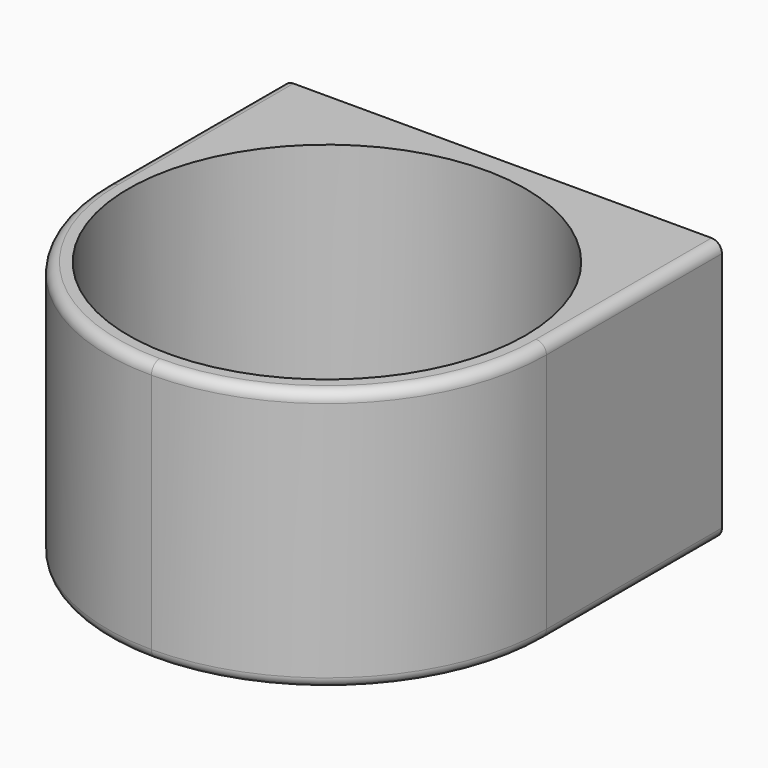
from build123d import *

# Parameters (mm, degrees)
F0_W     = 33.401
F0_H     = 33.401
F0_R     = 15.113
F1_DEPTH = 19.9644
F2_R     = 16.70049
F3_R     = 0.79375


# Not quite as in the source:
# - a fillet or chamfer is up to 0.001 mm smaller than in the source, because OpenCascade refuses the exact size


with BuildPart() as f1:
    # F0 (on Top) → F1 (new body)
    with BuildSketch(Plane.XY):
        Rectangle(F0_W, F0_H)
        Circle(F0_R, mode=Mode.SUBTRACT)
    extrude(amount=F1_DEPTH)

    # F2 (radius 16.7005 in the source; OpenCascade refuses exactly that, so slightly less here)
    f2_edges = [f1.edges().sort_by_distance(p)[0] for p in [
        (-16.7005, -16.7005, 9.9822),
        (16.7005, -16.7005, 9.9822),
    ]]
    fillet(f2_edges, radius=F2_R)

    # F3
    f3_edges = [f1.edges().sort_by_distance(p)[0] for p in [
        (11.80904, -11.80904, 19.9644),
        (11.80904, -11.80904, 0),
    ]]
    fillet(f3_edges, radius=F3_R)


solid = f1.part
